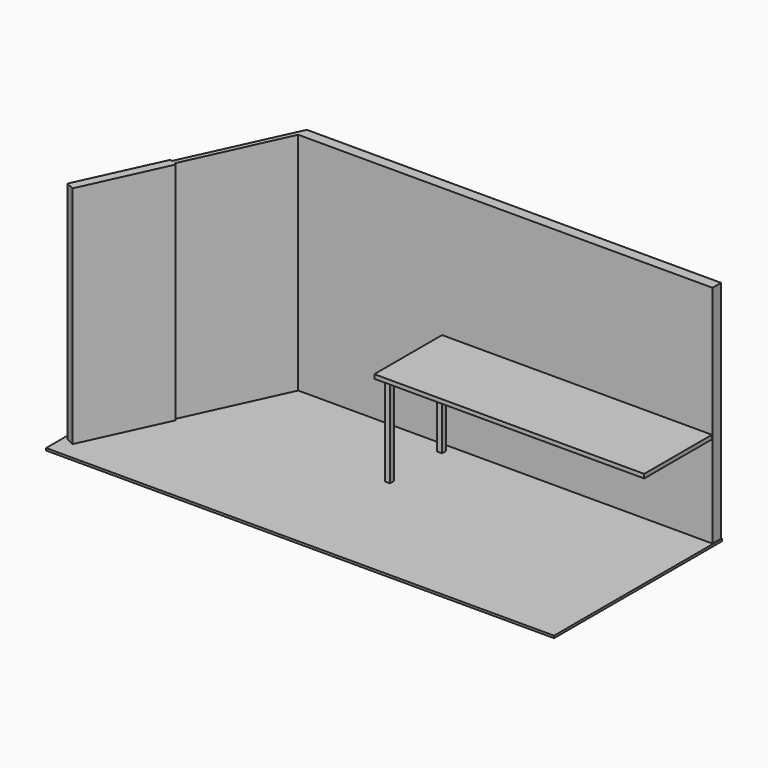
from build123d import *

# Parameters (mm, degrees)
F1_DEPTH = 2500
F3_W     = 2996.2194561958
F3_H     = 940.1818439364
F4_DEPTH = 45
F5_W     = 5639.598608017
F5_H     = 2329.9290537834
F6_DEPTH = 25
F7_W     = 55.7084493339
F7_H     = 55.7084493339
F8_DEPTH = 1020


with BuildPart() as f1:
    # F0 (on Top) → F1 (new body)
    with BuildSketch(Plane.XY):
        Polygon((-2237.7137064844, 864.2307190811), (-637.7137064844, 864.2307190811), (2362.2862935156, 864.2307190811), (2362.2862935156, 983.5458946084), (-2237.7137064844, 983.5458946084), (-2785.9814886635, -204.3676334463), (-2740.5835194385, -225.3205423194), align=None)
        Polygon((-2717.884534826, -235.796996756), (-2740.5835194385, -225.3205423194), (-2785.9814886635, -204.3676334463), (-2808.680473276, -193.8911790098), (-3227.7386507378, -1101.8505635102), (-3136.9427122877, -1143.7563812564), align=None)
    extrude(amount=F1_DEPTH)


with BuildPart() as f4:
    # F3 (on offset) → F4 (new body)
    with BuildSketch(Plane(origin=(0, 0, 1065), x_dir=(1, 0, 0), z_dir=(0, 0, -1))):
        with Locations((861.7163598537, -388.8723291457)):
            Rectangle(F3_W, F3_H)
    extrude(amount=F4_DEPTH)

    # F7 (on face) → F8 (join, through all)
    with BuildSketch(Plane(origin=(0, 0, 1020), x_dir=(1, 0, 0), z_dir=(0, 0, -1))):
        with Locations((-555.1630649716, -27.854224667)):
            Rectangle(F7_W, F7_H)
        with Locations((-555.1630649716, -749.8904336244)):
            Rectangle(F7_W, F7_H)
    extrude(amount=F8_DEPTH)


with BuildPart() as f6:
    # F5 (on face) → F6 (new body)
    with BuildSketch(Plane.XY):
        with Locations((-450.6896734238, -178.9979040623)):
            Rectangle(F5_W, F5_H)
        Polygon((-637.7137064844, 864.2307190811), (-2237.7137064844, 864.2307190811), (-2740.5835194385, -225.3205423194), (-2785.9814886635, -204.3676334463), (-2237.7137064844, 983.5458946084), (2362.2862935156, 983.5458946084), (2362.2862935156, 864.2307190811), align=None, mode=Mode.SUBTRACT)
    extrude(amount=-F6_DEPTH)


solid = Compound([f1.part, f4.part, f6.part])
